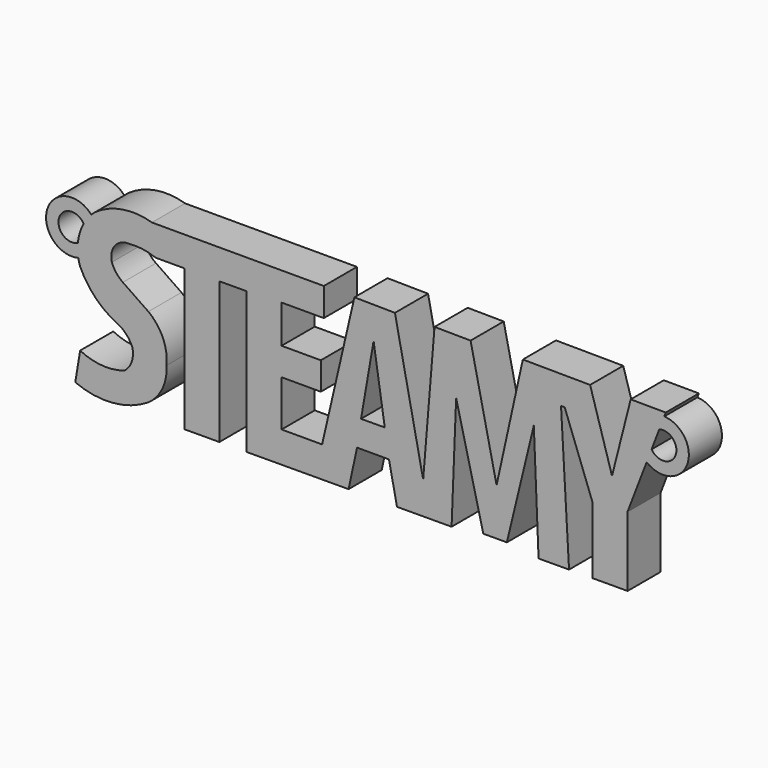
from build123d import *

# Parameters (mm, degrees)
F1_DEPTH = 5.08


# Not quite as in the source:
# - a feature names something its author has since deleted; it is built from what else it names


with BuildPart() as f1:
    # F0 (on Front) → F1 (new body)
    with BuildSketch(Plane.XZ):
        with BuildLine():
            Line((0.5275796089, 7.6204063303), (-20.5549836386, 7.6204063303))
            ThreePointArc((-20.5549836386, 7.6204063303), (-24.1470852619, 7.8573171504), (-27.4802406014, 6.4973920455))
            ThreePointArc((-27.4802406014, 6.4973920455), (-27.7375034402, 6.2746595983), (-27.981620644, 6.0375927257))
            ThreePointArc((-27.981620644, 6.0375927257), (-33.397838822, 4.8748506486), (-29.5783585742, 0.8624998257))
            ThreePointArc((-29.5783585742, 0.8624998257), (-29.4854309268, 0.4271699147), (-29.3602369053, 0))
            ThreePointArc((-29.3602369053, 0), (-27.3824789798, -2.8590960671), (-24.506347845, -4.8119981201))
            ThreePointArc((-24.506347845, -4.8119981201), (-23.6004229251, -5.5841706159), (-22.9712673668, -6.5946722771))
            ThreePointArc((-22.9712673668, -6.5946722771), (-23.0136087347, -8.1709506956), (-23.9121225745, -9.4667590625))
            ThreePointArc((-23.9121225745, -9.4667590625), (-26.6751520356, -9.8046566121), (-29.3602369053, -9.070609066))
            Line((-29.3602369053, -9.070609066), (-29.9534098835, -12.6854763365))
            ThreePointArc((-29.9534098835, -12.6854763365), (-25.3805938493, -13.4163192517), (-20.9905179357, -11.942544736))
            ThreePointArc((-20.9905179357, -11.942544736), (-19.2592379489, -9.8825014175), (-18.7621753773, -7.2378771215))
            ThreePointArc((-18.7621753773, -7.2378771215), (-19.211874139, -4.3971723931), (-20.9905179357, -2.1370266953))
            Line((-20.9905179357, -2.1370266953), (-24.1216853728, 0))
            ThreePointArc((-24.1216853728, 0), (-24.9307297161, 0.7590940477), (-25.4702806832, 1.7284553202))
            ThreePointArc((-25.4702806832, 1.7284553202), (-25.5043476571, 2.7102503227), (-25.1169531372, 3.6130279651))
            ThreePointArc((-25.1169531372, 3.6130279651), (-24.3175410864, 4.2333674235), (-23.3208688715, 4.4080819527))
            ThreePointArc((-23.3208688715, 4.4080819527), (-21.6899521733, 4.3761370029), (-20.1111126275, 3.9660450076))
            Line((-20.1111126275, 3.9660450076), (-16.5822823859, 3.9660450076))
            Line((-16.5822823859, 3.9660450076), (-16.5822823859, -13.4110949968))
            Line((-16.5822823859, -13.4110949968), (-12.2804131329, -13.3938708772))
            Line((-12.2804131329, -13.3938708772), (-12.2804131329, 3.9660450076))
            Line((-12.2804131329, 3.9660450076), (-8.945503985, 3.9793975459))
            Line((-8.945503985, 3.9793975459), (-8.945503985, -13.3805183388))
            Line((-8.945503985, -13.3805183388), (3.5631158198, -13.3304354676))
            Line((3.5631158198, -13.3304354676), (4.6038833267, -8.5034191039))
            Line((4.6038833267, -8.5034191039), (8.5180552324, -8.5034191039))
            Line((8.5180552324, -8.5034191039), (9.5034663795, -13.306651084))
            Line((9.5034663795, -13.306651084), (16.1975384964, -13.2798488983))
            Line((16.1975384964, -13.2798488983), (16.7558157547, 0.8041785421))
            Line((16.7558157547, 0.8041785421), (20.0938722411, -12.7696729569))
            Line((20.0938722411, -12.7696729569), (22.9795774261, -12.7581189723))
            Line((22.9795774261, -12.7581189723), (26.2847394813, 0.9427291897))
            Line((26.2847394813, 0.9427291897), (26.8666385735, -13.2371312225))
            Line((26.8666385735, -13.2371312225), (30.6037896767, -13.2221681602))
            Line((30.6037896767, -13.2221681602), (29.6197104597, 4.1383008359))
            Line((29.6197104597, 4.1383008359), (30.0681198915, 4.1383008359))
            Line((30.0681198915, 4.1383008359), (33.4722819544, -4.9878930799))
            Line((33.4722819544, -4.9878930799), (33.5052043981, -13.2105512767))
            Line((33.5052043981, -13.2105512767), (37.7860251854, -13.1934114324))
            Line((37.7860251854, -13.1934114324), (37.7674589547, -4.6679620266))
            Line((37.7674589547, -4.6679620266), (40.1194626421, 1.4735250723))
            ThreePointArc((40.1194626421, 1.4735250723), (45.0852633427, 2.8032642571), (42.2780045043, 7.1098499943))
            Line((42.2780045043, 7.1098499943), (42.4643497057, 7.59642944))
            Line((42.4643497057, 7.59642944), (38.1647445225, 7.6204063303))
            Line((38.1647445225, 7.6204063303), (35.8745108519, -1.3959297124))
            Line((35.8745108519, -1.3959297124), (33.1867010158, 7.5616615339))
            Line((33.1867010158, 7.5616615339), (24.9374744272, 7.6204063303))
            Line((24.9374744272, 7.6204063303), (21.7155495368, -7.0057700086))
            Line((21.7155495368, -7.0057700086), (18.5282991894, 7.5796761978))
            Line((18.5282991894, 7.5796761978), (14.1064790639, 7.6204063303))
            Line((14.1064790639, 7.6204063303), (12.7121774264, -9.3207750149))
            Line((12.7121774264, -9.3207750149), (9.2494001455, 7.5579893706))
            Line((9.2494001455, 7.5579893706), (4.2787034967, 7.6204063303))
            Line((4.2787034967, 7.6204063303), (0.3177259894, -9.5568800665))
            Line((0.3177259894, -9.5568800665), (-4.6531687161, -9.5568800665))
            Line((-4.6531687161, -9.5568800665), (-4.6531687161, -3.916612915))
            Line((-4.6531687161, -3.916612915), (0.1603365073, -3.916612915))
            Line((0.1603365073, -3.916612915), (0.1603365073, -0.5193359287))
            Line((0.1603365073, -0.5193359287), (-4.6531687161, -0.5193359287))
            Line((-4.6531687161, -0.5193359287), (-4.6531687161, 4.1502808179))
            Line((-4.6531687161, 4.1502808179), (0.5275796089, 4.1502808179))
            Line((0.5275796089, 4.1502808179), (0.5275796089, 7.6204063303))
        make_face()
        with BuildLine():
            ThreePointArc((-29.6399717805, 2.4549812242), (-31.9415802033, 4.4255324591), (-28.929800391, 4.7566757264))
            ThreePointArc((-28.929800391, 4.7566757264), (-29.4025078793, 3.6421198391), (-29.6399717805, 2.4549812242))
        make_face(mode=Mode.SUBTRACT)
        Polygon((8.0009574376, -5.2250216365), (5.0922911755, -5.2366675543), (6.6333247161, 3.6641330811), align=None, mode=Mode.SUBTRACT)
        with BuildLine():
            ThreePointArc((41.6721226179, 5.5277879385), (43.6620613807, 3.3483075355), (40.7253445285, 3.0555871281))
            Line((40.7253445285, 3.0555871281), (41.6721226179, 5.5277879385))
        make_face(mode=Mode.SUBTRACT)
    extrude(amount=F1_DEPTH)


solid = f1.part
